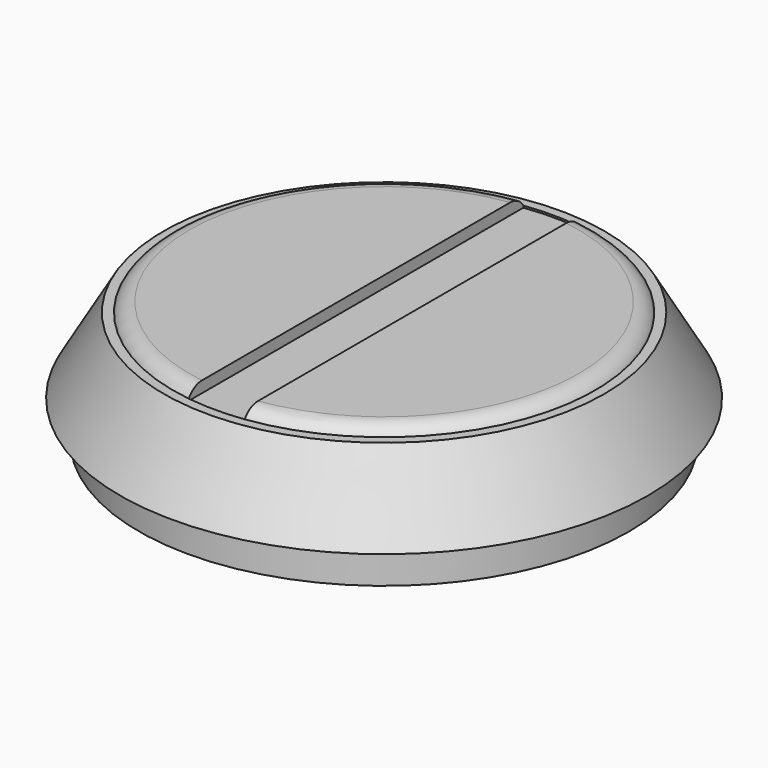
from build123d import *

# Parameters (mm, degrees)
F0_R     = 44.45
F0_R_2   = 41.275
F1_DEPTH = 12.7
F1_TAPER = 30
F2_DEPTH = 6.35
F3_R     = 35.5301515813
F4_DEPTH = 1.5875
F7_DEPTH = 2.9464
F8_DEPTH = 0.3175


# Not quite as in the source:
# - a fillet or chamfer that OpenCascade refuses, or shapes differently, is made with other operations: its cross-section is extruded or revolved along the edge and cut away or added


with BuildPart() as f1:
    # F0 (on Top) → F1 (new body)
    with BuildSketch(Plane.XY):
        Circle(F0_R)
        Circle(F0_R_2, mode=Mode.SUBTRACT)
        Circle(F0_R_2)
    extrude(amount=F1_DEPTH, taper=F1_TAPER)

    # F0 (on Top) → F2 (join)
    with BuildSketch(Plane.XY):
        Circle(F0_R_2)
    extrude(amount=-F2_DEPTH)

    # F3 (on face) → F4 (join)
    with BuildSketch(Plane.XY.offset(12.7)):
        Circle(F3_R)
    extrude(amount=F4_DEPTH)

    # F5: fillet of radius 3.175 on 1 edges, made by hand

    # F5_s1 → F5_t2 (revolve, cut)
    with BuildSketch(Plane.XZ):
        with BuildLine():
            ThreePointArc((35.5301515813, 12.7), (34.3680209243, 13.862130657), (32.7805209243, 14.2875))
            Line((32.7805209243, 14.2875), (35.5301515813, 14.2875))
            Line((35.5301515813, 14.2875), (35.5301515813, 12.7))
        make_face()
    revolve(axis=Axis((0, 0, 14.2875), (0, 0, 1)), mode=Mode.SUBTRACT)

    # F6 (on face) → F7 (cut)
    with BuildSketch(Plane.XY.offset(12.7)):
        with BuildLine():
            ThreePointArc((-4.7129914165, -35.0091413817), (0, -35.3249524893), (4.7129914165, -35.0091413817))
            Line((4.7129914165, -35.0091413817), (4.7129914165, 35.0091413817))
            ThreePointArc((4.7129914165, 35.0091413817), (0, 35.3249524893), (-4.7129914165, 35.0091413817))
            Line((-4.7129914165, 35.0091413817), (-4.7129914165, -35.0091413817))
        make_face()
        with BuildLine():
            ThreePointArc((-4.7129914165, -35.2161807029), (0, -35.5301515813), (4.7129914165, -35.2161807029))
            Line((4.7129914165, -35.2161807029), (4.7129914165, -35.0091413817))
            ThreePointArc((4.7129914165, -35.0091413817), (0, -35.3249524893), (-4.7129914165, -35.0091413817))
            Line((-4.7129914165, -35.0091413817), (-4.7129914165, -35.2161807029))
        make_face()
        with BuildLine():
            ThreePointArc((4.7129914165, 35.2161807029), (0, 35.5301515813), (-4.7129914165, 35.2161807029))
            Line((-4.7129914165, 35.2161807029), (-4.7129914165, 35.0091413817))
            ThreePointArc((-4.7129914165, 35.0091413817), (0, 35.3249524893), (4.7129914165, 35.0091413817))
            Line((4.7129914165, 35.0091413817), (4.7129914165, 35.2161807029))
        make_face()
    extrude(amount=F7_DEPTH, mode=Mode.SUBTRACT)

    # F6 (on face) → F8 (cut)
    with BuildSketch(Plane.XY.offset(12.7)):
        with BuildLine():
            ThreePointArc((-4.7129914165, -35.2161807029), (0, -35.5301515813), (4.7129914165, -35.2161807029))
            Line((4.7129914165, -35.2161807029), (4.7129914165, -35.0091413817))
            ThreePointArc((4.7129914165, -35.0091413817), (0, -35.3249524893), (-4.7129914165, -35.0091413817))
            Line((-4.7129914165, -35.0091413817), (-4.7129914165, -35.2161807029))
        make_face()
        with BuildLine():
            ThreePointArc((-4.7129914165, -35.0091413817), (0, -35.3249524893), (4.7129914165, -35.0091413817))
            Line((4.7129914165, -35.0091413817), (4.7129914165, 35.0091413817))
            ThreePointArc((4.7129914165, 35.0091413817), (0, 35.3249524893), (-4.7129914165, 35.0091413817))
            Line((-4.7129914165, 35.0091413817), (-4.7129914165, -35.0091413817))
        make_face()
        with BuildLine():
            ThreePointArc((4.7129914165, 35.2161807029), (0, 35.5301515813), (-4.7129914165, 35.2161807029))
            Line((-4.7129914165, 35.2161807029), (-4.7129914165, 35.0091413817))
            ThreePointArc((-4.7129914165, 35.0091413817), (0, 35.3249524893), (4.7129914165, 35.0091413817))
            Line((4.7129914165, 35.0091413817), (4.7129914165, 35.2161807029))
        make_face()
    extrude(amount=-F8_DEPTH, mode=Mode.SUBTRACT)


solid = f1.part
